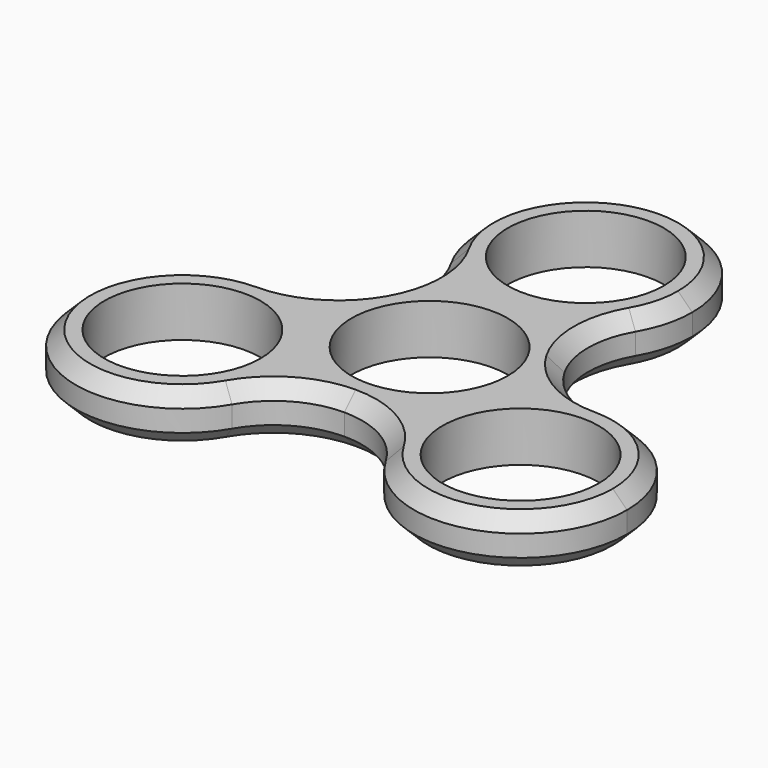
from build123d import *

# Parameters (mm, degrees)
F0_R     = 11
F1_DEPTH = 7
F2_R     = 12.499
F3_SIZE  = 2


# Not quite as in the source:
# - a fillet or chamfer is up to 0.001 mm smaller than in the source, because OpenCascade refuses the exact size


with BuildPart() as f1:
    # F0 (on Top) → F1 (new body)
    with BuildSketch(Plane.XY):
        with BuildLine():
            ThreePointArc((14.9052440041, -1.6833600857), (14.9762922658, -0.8430124372), (15, 0))
            ThreePointArc((15, 0), (12.5483433381, 8.2182163192), (5.9947894041, 13.75))
            ThreePointArc((5.9947894041, 13.75), (0, 12.5), (-5.9947894041, 13.75))
            ThreePointArc((-5.9947894041, 13.75), (-12.9903810568, 7.5), (-14.9052440041, -1.6833600857))
            ThreePointArc((-14.9052440041, -1.6833600857), (-10.8253175473, -6.25), (-8.9104546, -12.0666399143))
            ThreePointArc((-8.9104546, -12.0666399143), (0, -15), (8.9104546, -12.0666399143))
            ThreePointArc((8.9104546, -12.0666399143), (10.8253175473, -6.25), (14.9052440041, -1.6833600857))
        make_face()
        Circle(F0_R, mode=Mode.SUBTRACT)
        with BuildLine():
            ThreePointArc((-5.9947894041, 13.75), (0, 12.5), (5.9947894041, 13.75))
            ThreePointArc((5.9947894041, 13.75), (0, 15), (-5.9947894041, 13.75))
        make_face()
        with BuildLine():
            ThreePointArc((-5.9947894041, 13.75), (0, 15), (5.9947894041, 13.75))
            ThreePointArc((5.9947894041, 13.75), (12.5483433381, 19.2817836808), (15, 27.5))
            ThreePointArc((15, 27.5), (-8.2182163192, 40.0483433381), (-5.9947894041, 13.75))
        make_face()
        with Locations((0, 27.5)):
            Circle(F0_R, mode=Mode.SUBTRACT)
        with BuildLine():
            ThreePointArc((38.8156986041, -13.75), (30.5737745507, -0.3586442247), (14.9052440041, -1.6833600857))
            ThreePointArc((14.9052440041, -1.6833600857), (12.9903810568, -7.5), (8.9104546, -12.0666399143))
            ThreePointArc((8.9104546, -12.0666399143), (22.9726861669, -28.7262922658), (38.8156986041, -13.75))
        make_face()
        with Locations((23.8156986041, -13.75)):
            Circle(F0_R, mode=Mode.SUBTRACT)
        with BuildLine():
            ThreePointArc((8.9104546, -12.0666399143), (12.9903810568, -7.5), (14.9052440041, -1.6833600857))
            ThreePointArc((14.9052440041, -1.6833600857), (10.8253175473, -6.25), (8.9104546, -12.0666399143))
        make_face()
        with BuildLine():
            ThreePointArc((-8.9104546, -12.0666399143), (-10.8253175473, -6.25), (-14.9052440041, -1.6833600857))
            ThreePointArc((-14.9052440041, -1.6833600857), (-12.9903810568, -7.5), (-8.9104546, -12.0666399143))
        make_face()
        with BuildLine():
            ThreePointArc((-8.9104546, -12.0666399143), (-12.9903810568, -7.5), (-14.9052440041, -1.6833600857))
            ThreePointArc((-14.9052440041, -1.6833600857), (-37.2070543793, -20.5080759466), (-8.8156986041, -13.75))
            ThreePointArc((-8.8156986041, -13.75), (-8.8394063383, -12.9069875628), (-8.9104546, -12.0666399143))
        make_face()
        with Locations((-23.8156986041, -13.75)):
            Circle(F0_R, mode=Mode.SUBTRACT)
    extrude(amount=F1_DEPTH)

    # F2 (radius 12.5 in the source; OpenCascade refuses exactly that, so slightly less here)
    f2_edges = [f1.edges().sort_by_distance(p)[0] for p in [
        (-5.994789, 13.75, 3.5),
        (14.905244, -1.68336, 3.5),
        (-14.905244, -1.68336, 3.5),
        (5.994789, 13.75, 3.5),
        (-8.910455, -12.06664, 3.5),
        (8.910455, -12.06664, 3.5),
    ]]
    fillet(f2_edges, radius=F2_R)

    # F3
    f3_edges = [f1.edges().sort_by_distance(p)[0] for p in [
        (-6.250077, -16.674548, 0),
        (-6.250077, -16.674548, 7),
    ]]
    chamfer(f3_edges, length=F3_SIZE)


solid = f1.part
